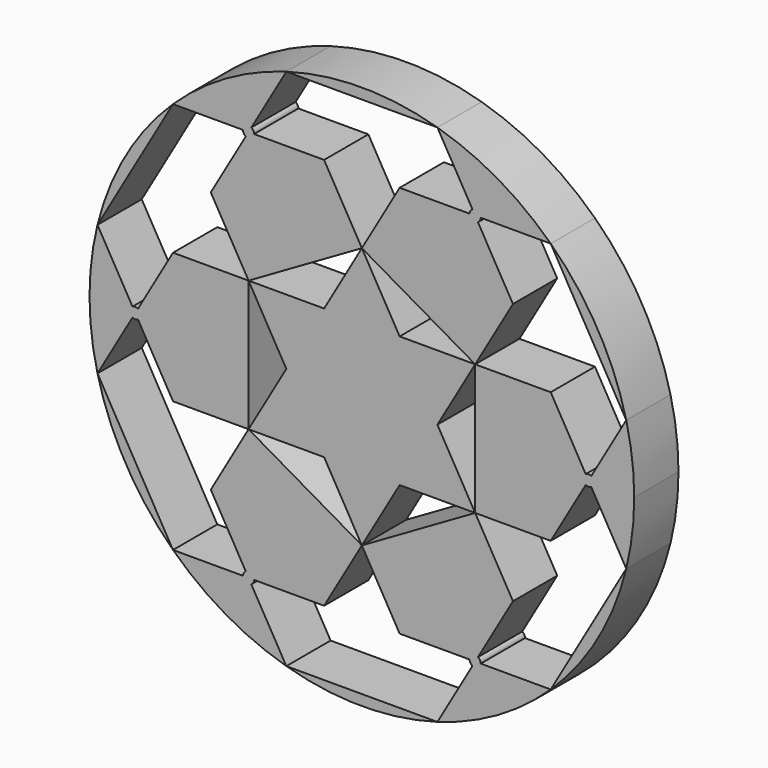
from build123d import *

# Parameters (mm, degrees)
F1_DEPTH = 6.35


# Not quite as in the source:
# - a feature names something its author has since deleted; it is built from what else it names


with BuildPart() as f1:
    # F0 (on Front) → F1 (new body)
    with BuildSketch(Plane.XZ):
        with BuildLine():
            Line((21.6713532185, 7.5071769686), (13.0028119311, 7.5071769686))
            Line((13.0028119311, 7.5071769686), (13.0028119311, -7.5071769686))
            Line((13.0028119311, -7.5071769686), (21.6713532185, -7.5071769686))
            Line((21.6713532185, -7.5071769686), (25.6881238621, -0.5499261314))
            ThreePointArc((25.6881238621, -0.5499261314), (25.3706238621, 0), (25.6881238621, 0.5499261314))
            Line((25.6881238621, 0.5499261314), (21.6713532185, 7.5071769686))
        make_face()
        with BuildLine():
            ThreePointArc((26.3231238621, 0.5499261314), (26.0056238621, 0.635), (25.6881238621, 0.5499261314))
            ThreePointArc((25.6881238621, 0.5499261314), (25.3706238621, 0), (25.6881238621, -0.5499261314))
            ThreePointArc((25.6881238621, -0.5499261314), (26.0056238621, -0.635), (26.3231238621, -0.5499261314))
            ThreePointArc((26.3231238621, -0.5499261314), (26.5555499936, -0.3175), (26.6406238621, 0))
            ThreePointArc((26.6406238621, 0), (26.5555499936, 0.3175), (26.3231238621, 0.5499261314))
        make_face()
        with BuildLine():
            Line((30.3398945058, 7.5071769686), (26.3231238621, 0.5499261314))
            ThreePointArc((26.3231238621, 0.5499261314), (26.5555499936, 0.3175), (26.6406238621, 0))
            ThreePointArc((26.6406238621, 0), (26.5555499936, -0.3175), (26.3231238621, -0.5499261314))
            Line((26.3231238621, -0.5499261314), (30.3398945058, -7.5071769686))
            ThreePointArc((30.3398945058, -7.5071769686), (31.0252829652, -3.7813650434), (31.2548700951, 0))
            ThreePointArc((31.2548700951, 0), (31.0252829652, 3.7813650434), (30.3398945058, 7.5071769686))
        make_face()
    extrude(amount=F1_DEPTH)


with BuildPart() as f1b:
    # F0 (on Front) → F1, piece 2 (new body)
    with BuildSketch(Plane.XZ):
        with BuildLine():
            Line((0, 15.0143539373), (13.0028119311, 7.5071769686))
            Line((13.0028119311, 7.5071769686), (17.3370825748, 15.0143539373))
            Line((17.3370825748, 15.0143539373), (13.3203119311, 21.9716047745))
            ThreePointArc((13.3203119311, 21.9716047745), (12.6853119311, 21.9716047745), (12.3678119311, 22.5215309059))
            Line((12.3678119311, 22.5215309059), (4.3342706437, 22.5215309059))
            Line((4.3342706437, 22.5215309059), (0, 15.0143539373))
        make_face()
        with BuildLine():
            ThreePointArc((12.3678119311, 22.5215309059), (12.6853119311, 21.9716047745), (13.3203119311, 21.9716047745))
            ThreePointArc((13.3203119311, 21.9716047745), (13.5527380625, 22.2040309059), (13.6378119311, 22.5215309059))
            ThreePointArc((13.6378119311, 22.5215309059), (13.3203119311, 23.0714570373), (12.6853119311, 23.0714570373))
            ThreePointArc((12.6853119311, 23.0714570373), (12.4528857997, 22.8390309059), (12.3678119311, 22.5215309059))
        make_face()
        with BuildLine():
            ThreePointArc((12.6853119311, 23.0714570373), (13.3203119311, 23.0714570373), (13.6378119311, 22.5215309059))
            Line((13.6378119311, 22.5215309059), (21.6713532185, 22.5215309059))
            ThreePointArc((21.6713532185, 22.5215309059), (15.6274350476, 27.0675114944), (8.6685412874, 30.0287078745))
            Line((8.6685412874, 30.0287078745), (12.6853119311, 23.0714570373))
        make_face()
    extrude(amount=F1_DEPTH)


with BuildPart() as f1c:
    # F0 (on Front) → F1, piece 3 (new body)
    with BuildSketch(Plane.XZ):
        Polygon((8.6685412874, 0), (13.0028119311, 7.5071769686), (4.3342706437, 7.5071769686), (0, 0), align=None)
        Polygon((4.3342706437, -7.5071769686), (13.0028119311, -7.5071769686), (8.6685412874, 0), (0, 0), align=None)
        Polygon((4.3342706437, 7.5071769686), (0, 15.0143539373), (-4.3342706437, 7.5071769686), (0, 0), align=None)
        Polygon((-4.3342706437, -7.5071769686), (0, -15.0143539373), (4.3342706437, -7.5071769686), (0, 0), align=None)
        Polygon((-4.3342706437, 7.5071769686), (-13.0028119311, 7.5071769686), (-8.6685412874, 0), (0, 0), align=None)
        Polygon((-4.3342706437, -7.5071769686), (0, 0), (-8.6685412874, 0), (-13.0028119311, -7.5071769686), align=None)
    extrude(amount=F1_DEPTH)


with BuildPart() as f1d:
    # F0 (on Front) → F1, piece 4 (new body)
    with BuildSketch(Plane.XZ):
        with BuildLine():
            Line((17.3370825748, -15.0143539373), (13.0028119311, -7.5071769686))
            Line((13.0028119311, -7.5071769686), (0, -15.0143539373))
            Line((0, -15.0143539373), (4.3342706437, -22.5215309059))
            Line((4.3342706437, -22.5215309059), (12.3678119311, -22.5215309059))
            ThreePointArc((12.3678119311, -22.5215309059), (12.6853119311, -21.9716047745), (13.3203119311, -21.9716047745))
            Line((13.3203119311, -21.9716047745), (17.3370825748, -15.0143539373))
        make_face()
        with BuildLine():
            ThreePointArc((13.6378119311, -22.5215309059), (13.5527380625, -22.2040309059), (13.3203119311, -21.9716047745))
            ThreePointArc((13.3203119311, -21.9716047745), (12.6853119311, -21.9716047745), (12.3678119311, -22.5215309059))
            ThreePointArc((12.3678119311, -22.5215309059), (12.4528857997, -22.8390309059), (12.6853119311, -23.0714570373))
            ThreePointArc((12.6853119311, -23.0714570373), (13.3203119311, -23.0714570373), (13.6378119311, -22.5215309059))
        make_face()
        with BuildLine():
            Line((21.6713532185, -22.5215309059), (13.6378119311, -22.5215309059))
            ThreePointArc((13.6378119311, -22.5215309059), (13.3203119311, -23.0714570373), (12.6853119311, -23.0714570373))
            Line((12.6853119311, -23.0714570373), (8.6685412874, -30.0287078745))
            ThreePointArc((8.6685412874, -30.0287078745), (15.6274350476, -27.0675114944), (21.6713532185, -22.5215309059))
        make_face()
    extrude(amount=F1_DEPTH)


with BuildPart() as f1e:
    # F0 (on Front) → F1, piece 5 (new body)
    with BuildSketch(Plane.XZ):
        with BuildLine():
            Line((-13.0028119311, 7.5071769686), (0, 15.0143539373))
            Line((0, 15.0143539373), (-4.3342706437, 22.5215309059))
            Line((-4.3342706437, 22.5215309059), (-12.3678119311, 22.5215309059))
            ThreePointArc((-12.3678119311, 22.5215309059), (-12.6853119311, 21.9716047745), (-13.3203119311, 21.9716047745))
            Line((-13.3203119311, 21.9716047745), (-17.3370825748, 15.0143539373))
            Line((-17.3370825748, 15.0143539373), (-13.0028119311, 7.5071769686))
        make_face()
        with BuildLine():
            ThreePointArc((-13.3203119311, 21.9716047745), (-12.6853119311, 21.9716047745), (-12.3678119311, 22.5215309059))
            ThreePointArc((-12.3678119311, 22.5215309059), (-12.4528857997, 22.8390309059), (-12.6853119311, 23.0714570373))
            ThreePointArc((-12.6853119311, 23.0714570373), (-13.3203119311, 23.0714570373), (-13.6378119311, 22.5215309059))
            ThreePointArc((-13.6378119311, 22.5215309059), (-13.5527380625, 22.2040309059), (-13.3203119311, 21.9716047745))
        make_face()
        with BuildLine():
            ThreePointArc((-13.6378119311, 22.5215309059), (-13.3203119311, 23.0714570373), (-12.6853119311, 23.0714570373))
            Line((-12.6853119311, 23.0714570373), (-8.6685412874, 30.0287078745))
            ThreePointArc((-8.6685412874, 30.0287078745), (-15.6274350476, 27.0675114944), (-21.6713532185, 22.5215309059))
            Line((-21.6713532185, 22.5215309059), (-13.6378119311, 22.5215309059))
        make_face()
    extrude(amount=F1_DEPTH)


with BuildPart() as f1f:
    # F0 (on Front) → F1, piece 6 (new body)
    with BuildSketch(Plane.XZ):
        with BuildLine():
            Line((-4.3342706437, -22.5215309059), (0, -15.0143539373))
            Line((0, -15.0143539373), (-13.0028119311, -7.5071769686))
            Line((-13.0028119311, -7.5071769686), (-17.3370825748, -15.0143539373))
            Line((-17.3370825748, -15.0143539373), (-13.3203119311, -21.9716047745))
            ThreePointArc((-13.3203119311, -21.9716047745), (-12.6853119311, -21.9716047745), (-12.3678119311, -22.5215309059))
            Line((-12.3678119311, -22.5215309059), (-4.3342706437, -22.5215309059))
        make_face()
        with BuildLine():
            ThreePointArc((-12.6853119311, -23.0714570373), (-12.4528857997, -22.8390309059), (-12.3678119311, -22.5215309059))
            ThreePointArc((-12.3678119311, -22.5215309059), (-12.6853119311, -21.9716047745), (-13.3203119311, -21.9716047745))
            ThreePointArc((-13.3203119311, -21.9716047745), (-13.5527380625, -22.2040309059), (-13.6378119311, -22.5215309059))
            ThreePointArc((-13.6378119311, -22.5215309059), (-13.3203119311, -23.0714570373), (-12.6853119311, -23.0714570373))
        make_face()
        with BuildLine():
            Line((-8.6685412874, -30.0287078745), (-12.6853119311, -23.0714570373))
            ThreePointArc((-12.6853119311, -23.0714570373), (-13.3203119311, -23.0714570373), (-13.6378119311, -22.5215309059))
            Line((-13.6378119311, -22.5215309059), (-21.6713532185, -22.5215309059))
            ThreePointArc((-21.6713532185, -22.5215309059), (-15.6274350476, -27.0675114944), (-8.6685412874, -30.0287078745))
        make_face()
    extrude(amount=F1_DEPTH)


with BuildPart() as f1g:
    # F0 (on Front) → F1, piece 7 (new body)
    with BuildSketch(Plane.XZ):
        with BuildLine():
            Line((-13.0028119311, -7.5071769686), (-13.0028119311, 7.5071769686))
            Line((-13.0028119311, 7.5071769686), (-21.6713532185, 7.5071769686))
            Line((-21.6713532185, 7.5071769686), (-25.6881238621, 0.5499261314))
            ThreePointArc((-25.6881238621, 0.5499261314), (-25.4556977307, 0.3175), (-25.3706238621, 0))
            ThreePointArc((-25.3706238621, 0), (-25.4556977307, -0.3175), (-25.6881238621, -0.5499261314))
            Line((-25.6881238621, -0.5499261314), (-21.6713532185, -7.5071769686))
            Line((-21.6713532185, -7.5071769686), (-13.0028119311, -7.5071769686))
        make_face()
        with BuildLine():
            ThreePointArc((-25.3706238621, 0), (-25.4556977307, 0.3175), (-25.6881238621, 0.5499261314))
            ThreePointArc((-25.6881238621, 0.5499261314), (-26.0056238621, 0.635), (-26.3231238621, 0.5499261314))
            ThreePointArc((-26.3231238621, 0.5499261314), (-26.6406238621, 0), (-26.3231238621, -0.5499261314))
            ThreePointArc((-26.3231238621, -0.5499261314), (-26.0056238621, -0.635), (-25.6881238621, -0.5499261314))
            ThreePointArc((-25.6881238621, -0.5499261314), (-25.4556977307, -0.3175), (-25.3706238621, 0))
        make_face()
        with BuildLine():
            ThreePointArc((-26.3231238621, -0.5499261314), (-26.6406238621, 0), (-26.3231238621, 0.5499261314))
            Line((-26.3231238621, 0.5499261314), (-30.3398945058, 7.5071769686))
            ThreePointArc((-30.3398945058, 7.5071769686), (-31.2548700951, 0), (-30.3398945058, -7.5071769686))
            Line((-30.3398945058, -7.5071769686), (-26.3231238621, -0.5499261314))
        make_face()
    extrude(amount=F1_DEPTH)


with BuildPart() as f1h:
    # F0 (on Front) → F1, piece 8 (new body)
    with BuildSketch(Plane.XZ):
        with BuildLine():
            ThreePointArc((30.3398945058, 7.5071769686), (27.0675114944, 15.6274350476), (21.6713532185, 22.5215309059))
            Line((21.6713532185, 22.5215309059), (30.3398945058, 7.5071769686))
        make_face()
    extrude(amount=F1_DEPTH)


with BuildPart() as f1i:
    # F0 (on Front) → F1, piece 9 (new body)
    with BuildSketch(Plane.XZ):
        with BuildLine():
            Line((30.3398945058, -7.5071769686), (21.6713532185, -22.5215309059))
            ThreePointArc((21.6713532185, -22.5215309059), (27.0675114944, -15.6274350476), (30.3398945058, -7.5071769686))
        make_face()
    extrude(amount=F1_DEPTH)


with BuildPart() as f1j:
    # F0 (on Front) → F1, piece 10 (new body)
    with BuildSketch(Plane.XZ):
        with BuildLine():
            ThreePointArc((8.6685412874, 30.0287078745), (0, 31.2548700951), (-8.6685412874, 30.0287078745))
            Line((-8.6685412874, 30.0287078745), (8.6685412874, 30.0287078745))
        make_face()
    extrude(amount=F1_DEPTH)


with BuildPart() as f1k:
    # F0 (on Front) → F1, piece 11 (new body)
    with BuildSketch(Plane.XZ):
        with BuildLine():
            ThreePointArc((-8.6685412874, -30.0287078745), (0, -31.2548700951), (8.6685412874, -30.0287078745))
            Line((8.6685412874, -30.0287078745), (-8.6685412874, -30.0287078745))
        make_face()
    extrude(amount=F1_DEPTH)


with BuildPart() as f1l:
    # F0 (on Front) → F1, piece 12 (new body)
    with BuildSketch(Plane.XZ):
        with BuildLine():
            Line((-30.3398945058, 7.5071769686), (-21.6713532185, 22.5215309059))
            ThreePointArc((-21.6713532185, 22.5215309059), (-27.0675114944, 15.6274350476), (-30.3398945058, 7.5071769686))
        make_face()
    extrude(amount=F1_DEPTH)


with BuildPart() as f1m:
    # F0 (on Front) → F1, piece 13 (new body)
    with BuildSketch(Plane.XZ):
        with BuildLine():
            ThreePointArc((-30.3398945058, -7.5071769686), (-27.0675114944, -15.6274350476), (-21.6713532185, -22.5215309059))
            Line((-21.6713532185, -22.5215309059), (-30.3398945058, -7.5071769686))
        make_face()
    extrude(amount=F1_DEPTH)


solid = Compound([f1.part, f1b.part, f1c.part, f1d.part, f1e.part, f1f.part, f1g.part, f1h.part, f1i.part, f1j.part, f1k.part, f1l.part, f1m.part])
